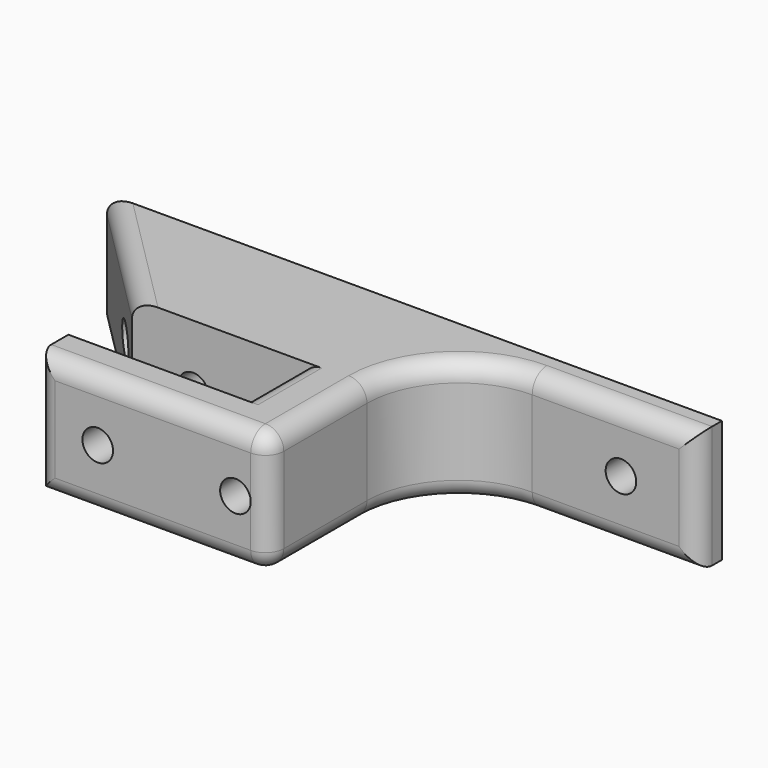
from build123d import *

# Parameters (mm, degrees)
F1_DEPTH = 20
F2_R     = 2.5
F3_DEPTH = 50
F4_R     = 2.99999


# Not quite as in the source:
# - a fillet or chamfer is up to 0.001 mm smaller than in the source, because OpenCascade refuses the exact size


with BuildPart() as f1:
    # F0 (on Top) → F1 (new body)
    with BuildSketch(Plane.XY):
        with BuildLine():
            Line((80, 0), (-20.5, 0))
            Line((-20.5, 0), (0, -20.5))
            Line((0, -20.5), (28, -20.5))
            Line((28, -20.5), (28, -33.5))
            Line((28, -33.5), (0, -33.5))
            Line((0, -33.5), (0, -40))
            Line((0, -40), (38, -40))
            Line((38, -40), (38, -20))
            ThreePointArc((38, -20), (42.3933982822, -9.3933982822), (53, -5))
            Line((53, -5), (80, -5))
            Line((80, -5), (80, 0))
        make_face()
    extrude(amount=F1_DEPTH)

    # F2 (on Front) → F3 (cut)
    with BuildSketch(Plane.XZ):
        with Locations((10, 10)):
            Circle(F2_R)
        with Locations((-5.5, 10)):
            Circle(F2_R)
        with Locations((32.5, 10)):
            Circle(F2_R)
        with Locations((67.5, 10)):
            Circle(F2_R)
    extrude(amount=F3_DEPTH, mode=Mode.SUBTRACT)

    # F4 (radius 3 in the source; OpenCascade refuses exactly that, so slightly less here)
    f4_edges = [f1.edges().sort_by_distance(p)[0] for p in [
        (66.5, -5, 20),
        (19, -40, 20),
        (0, -40, 10),
        (19, -40, 0),
        (66.5, -5, 0),
        (-10.25, -10.25, 20),
        (-10.25, -10.25, 0),
        (80, -5, 10),
        (38, -40, 10),
        (28, -27, 20),
        (28, -27, 0),
    ]]
    fillet(f4_edges, radius=F4_R)


solid = f1.part
